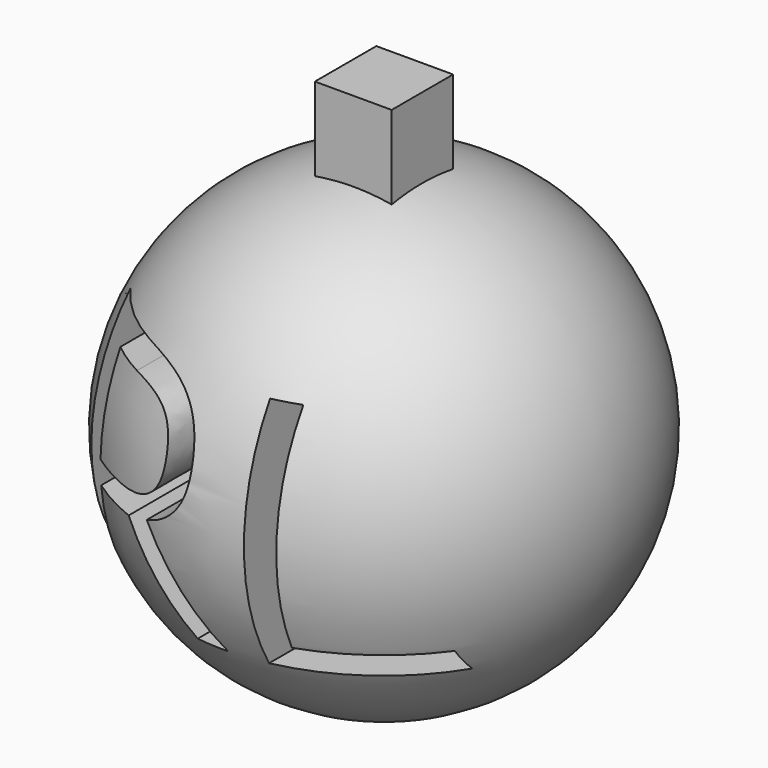
from build123d import *

# Parameters (mm, degrees)
F3_W         = 12.7
F3_H         = 12.7
F4_DEPTH     = 25.4
F5_TEXT_SIZE = 53.8563477339
F6_DEPTH     = 101.6
F7_W         = 7.2292946279
F7_H         = 14.570672065
F8_DEPTH     = 12.7


# Not quite as in the source:
# - Text() gives the source's letters only with a copy of the font that has no kerning and outlines rounded to 1/6400 em; it was checked with that copy


with BuildPart() as f1:
    # F0 (on Front) → F1 (revolve)
    with BuildSketch(Plane.XZ):
        with BuildLine():
            Line((0, 76.2), (0, 0))
            ThreePointArc((0, 0), (38.1, 38.1), (0, 76.2))
        make_face()
    revolve(axis=Axis((0, 0, 38.1), (0, 0, 1)))

    # F3 (on offset) → F4 (join)
    with BuildSketch(Plane.XY.offset(88.9)):
        Rectangle(F3_W, F3_H)
    extrude(amount=-F4_DEPTH)

    # F5 (on Front) → F6 (cut, symmetric)
    with BuildSketch(Plane.XZ):
        with Locations((-31.75, 19.05)):
            Text('RL', F5_TEXT_SIZE, font='Open Sans', text_align=(TextAlign.LEFT, TextAlign.BOTTOM))
    extrude(amount=F6_DEPTH, both=True, mode=Mode.SUBTRACT)

    # F7 (on Front) → F8 (join)
    with BuildSketch(Plane.XZ):
        with Locations((-25.0884164125, 46.2394040078)):
            Rectangle(F7_W, F7_H)
    extrude(amount=F8_DEPTH)


solid = f1.part
